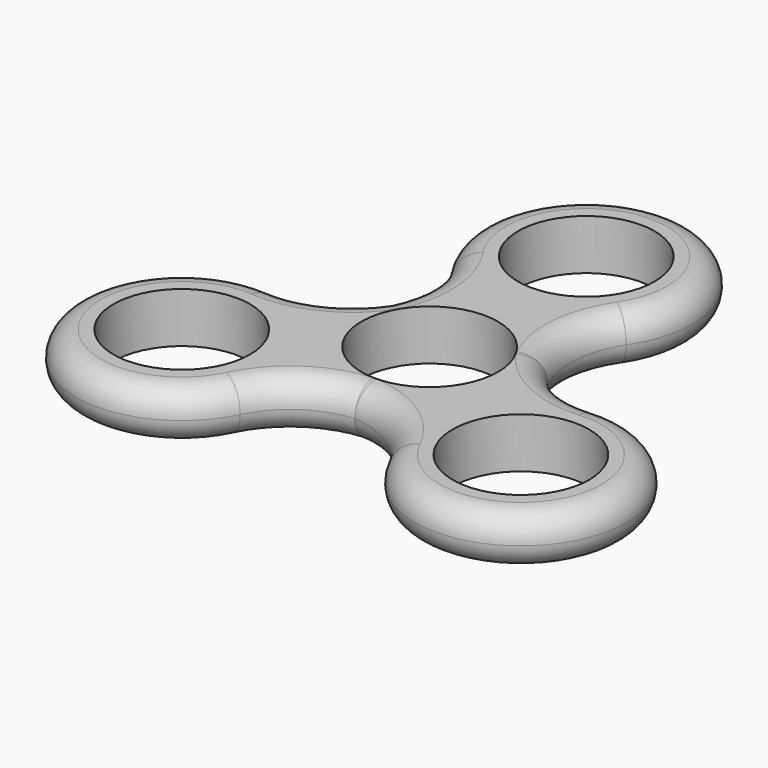
from build123d import *

# Parameters (mm, degrees)
F1_DEPTH = 7.112
F2_R     = 3.556
F2_R_2   = 3.55599
F3_R     = 9.652
F4_DEPTH = 7.1130001


# Not quite as in the source:
# - a fillet or chamfer is up to 0.001 mm smaller than in the source, because OpenCascade refuses the exact size


with BuildPart() as f1:
    # F0 (on Top) → F1 (new body)
    with BuildSketch(Plane.XY):
        with BuildLine():
            ThreePointArc((11.4542066283, 6.6130892802), (10.2320494736, 13.0629936143), (12.3938687373, 19.2614992004))
            ThreePointArc((12.3938687373, 19.2614992004), (0, 42.672), (-12.3938687373, 19.2614992004))
            ThreePointArc((-12.3938687373, 19.2614992004), (-10.2320494736, 13.0629936143), (-11.4542066283, 6.6130892802))
            ThreePointArc((-11.4542066283, 6.6130892802), (-16.4289090562, 2.3297179697), (-22.8778819912, 1.1026555775))
            ThreePointArc((-22.8778819912, 1.1026555775), (-36.9550360303, -21.336), (-10.4840132539, -20.3641547779))
            ThreePointArc((-10.4840132539, -20.3641547779), (-6.1968595827, -15.392711584), (0, -13.2261785604))
            ThreePointArc((0, -13.2261785604), (6.1968595827, -15.392711584), (10.4840132539, -20.3641547779))
            ThreePointArc((10.4840132539, -20.3641547779), (36.9550360303, -21.336), (22.8778819912, 1.1026555775))
            ThreePointArc((22.8778819912, 1.1026555775), (16.4289090562, 2.3297179697), (11.4542066283, 6.6130892802))
        make_face()
        with BuildLine():
            ThreePointArc((-11.6730555007, 6.1798899083), (-11.5615614887, 6.395444061), (-11.4542066283, 6.6130892802))
            ThreePointArc((-11.4542066283, 6.6130892802), (-11.3193977697, 6.8148839261), (-11.1884694035, 7.0192176492))
            ThreePointArc((-11.1884694035, 7.0192176492), (-11.4384635332, 6.604), (-11.6730555007, 6.1798899083))
        make_face(mode=Mode.SUBTRACT)
        with BuildLine():
            ThreePointArc((0.4845860972, -13.1991075575), (0.242163719, -13.2103279872), (0, -13.2261785604))
            ThreePointArc((0, -13.2261785604), (-0.242163719, -13.2103279872), (-0.4845860972, -13.1991075575))
            ThreePointArc((-0.4845860972, -13.1991075575), (0, -13.208), (0.4845860972, -13.1991075575))
        make_face(mode=Mode.SUBTRACT)
        with BuildLine():
            ThreePointArc((11.1884694035, 7.0192176492), (11.3193977697, 6.8148839261), (11.4542066283, 6.6130892802))
            ThreePointArc((11.4542066283, 6.6130892802), (11.5615614887, 6.395444061), (11.6730555007, 6.1798899083))
            ThreePointArc((11.6730555007, 6.1798899083), (11.4384635332, 6.604), (11.1884694035, 7.0192176492))
        make_face(mode=Mode.SUBTRACT)
        with BuildLine():
            ThreePointArc((-11.1884694035, 7.0192176492), (-11.3193977697, 6.8148839261), (-11.4542066283, 6.6130892802))
            ThreePointArc((-11.4542066283, 6.6130892802), (-11.5615614887, 6.395444061), (-11.6730555007, 6.1798899083))
            ThreePointArc((-11.6730555007, 6.1798899083), (-11.4384635332, 6.604), (-11.1884694035, 7.0192176492))
        make_face()
        with BuildLine():
            ThreePointArc((-0.4845860972, -13.1991075575), (-0.242163719, -13.2103279872), (0, -13.2261785604))
            ThreePointArc((0, -13.2261785604), (0.242163719, -13.2103279872), (0.4845860972, -13.1991075575))
            ThreePointArc((0.4845860972, -13.1991075575), (0, -13.208), (-0.4845860972, -13.1991075575))
        make_face()
        with BuildLine():
            ThreePointArc((11.6730555007, 6.1798899083), (11.5615614887, 6.395444061), (11.4542066283, 6.6130892802))
            ThreePointArc((11.4542066283, 6.6130892802), (11.3193977697, 6.8148839261), (11.1884694035, 7.0192176492))
            ThreePointArc((11.1884694035, 7.0192176492), (11.4384635332, 6.604), (11.6730555007, 6.1798899083))
        make_face()
    extrude(amount=F1_DEPTH)

    # F2 (call 1 of 2: OpenCascade refuses the feature's edges together)
    f2_edges = [f1.edges().sort_by_distance(p)[0] for p in [
        (-6.19686, -15.392712, 7.112),
        (6.19686, -15.392712, 7.112),
        (36.955036, -21.336, 7.112),
        (16.428909, 2.329718, 7.112),
        (10.232049, 13.062994, 7.112),
        (0, 42.672, 7.112),
        (-10.232049, 13.062994, 7.112),
        (-16.428909, 2.329718, 7.112),
        (-36.955036, -21.336, 7.112),
    ]]
    fillet(f2_edges, radius=F2_R)

    # F2#2 (call 2 of 2) (radius 3.556 in the source; OpenCascade refuses exactly that, so slightly less here)
    f2_2_edges = [f1.edges().sort_by_distance(p)[0] for p in [
        (-6.19686, -15.392712, 0),
        (6.19686, -15.392712, 0),
        (36.955036, -21.336, 0),
        (16.428909, 2.329718, 0),
        (10.232049, 13.062994, 0),
        (0, 42.672, 0),
        (-10.232049, 13.062994, 0),
        (-16.428909, 2.329718, 0),
        (-36.955036, -21.336, 0),
    ]]
    fillet(f2_2_edges, radius=F2_R_2)

    # F3 (on face) → F4 (cut, through all)
    with BuildSketch(Plane.XY.offset(7.112)):
        with Locations((-1.06793e-05, 0)):
            Circle(F3_R)
        with Locations((0, 27.686)):
            Circle(F3_R)
        with Locations((-23.9767793292, -13.843)):
            Circle(F3_R)
        with Locations((23.9767793292, -13.843)):
            Circle(F3_R)
    extrude(amount=-F4_DEPTH, mode=Mode.SUBTRACT)


solid = f1.part
